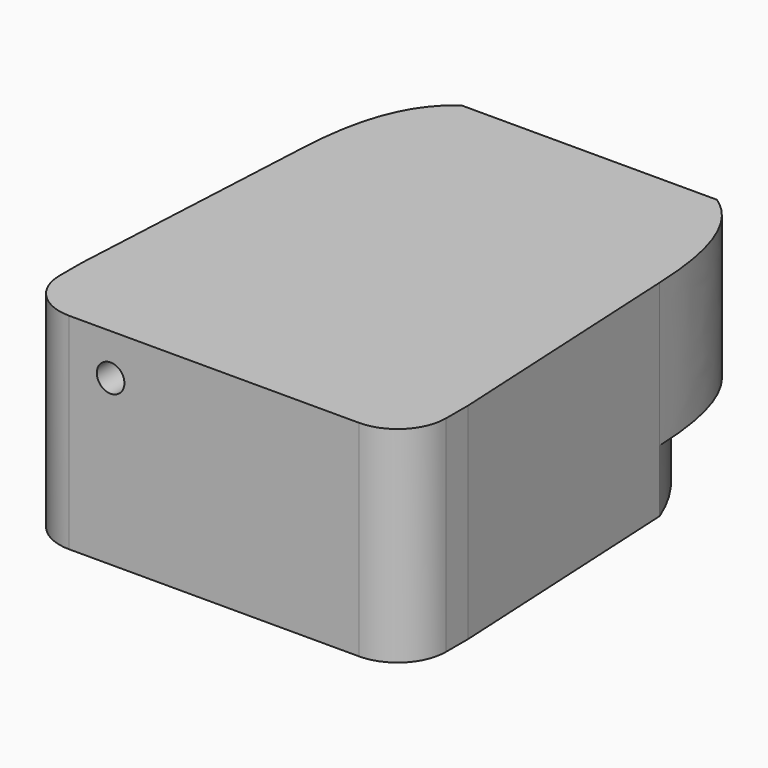
from build123d import *

# Parameters (mm, degrees)
F1_DEPTH  = 4.5
F3_DEPTH  = 10.4
F5_DEPTH  = 13.4
F6_R      = 3.7
F6_R_2    = 1.6
F7_DEPTH  = 5
F8_R      = 1.6
F8_R_2    = 3.7
F9_DEPTH  = 5
F10_R     = 1
F11_DEPTH = 2
F12_W     = 10
F12_H     = 1.5
F13_DEPTH = 3


with BuildPart() as f1:
    # F0 (on Top) → F1 (new body)
    with BuildSketch(Plane.XY):
        with BuildLine():
            ThreePointArc((-14, -13.8007847667), (-12.9748737342, -16.2756585008), (-10.5, -17.3007847667))
            Line((-10.5, -17.3007847667), (-6.75, -17.3007847667))
            Line((-6.75, -17.3007847667), (6.75, -17.3007847667))
            Line((6.75, -17.3007847667), (10.5, -17.3007847667))
            ThreePointArc((10.5, -17.3007847667), (12.9748737342, -16.2756585008), (14, -13.8007847667))
            Line((14, -13.8007847667), (14, -11.8007847667))
            Line((14, -11.8007847667), (13.0486556537, 6.7504299853))
            ThreePointArc((13.0486556537, 6.7504299853), (11.6774697173, 9.4001806183), (9.7759521317, 11.6992152333))
            Line((9.7759521317, 11.6992152333), (-9.7759521317, 11.6992152333))
            ThreePointArc((-9.7759521317, 11.6992152333), (-11.6774697173, 9.4001806183), (-13.0486556537, 6.7504299853))
            Line((-13.0486556537, 6.7504299853), (-14, -11.8007847667))
            Line((-14, -11.8007847667), (-14, -13.8007847667))
        make_face()
    extrude(amount=F1_DEPTH)

    # F2 (on face) → F3 (join)
    with BuildSketch(Plane.XY.offset(4.5)):
        with BuildLine():
            Line((14, -13.8007847667), (14, -11.8007847667))
            Line((14, -11.8007847667), (13.0486556537, 6.7504299853))
            add(Edge.make_bspline(
                [(13.0486556537, 6.7504299853), (12.8450421616, 12.0132155716), (11.5178218111, 15.1653625071), (9.2356767608, 16.6992152333)],
                knots=[0, 0, 0, 0, 10.6544420759, 10.6544420759, 10.6544420759, 10.6544420759], degree=3))
            Line((9.2356767608, 16.6992152333), (-9.2356767608, 16.6992152333))
            add(Edge.make_bspline(
                [(-13.0486556537, 6.7504299853), (-12.8450421616, 12.0132155716), (-11.5178218111, 15.1653625071), (-9.2356767608, 16.6992152333)],
                knots=[0, 0, 0, 0, 10.6544420759, 10.6544420759, 10.6544420759, 10.6544420759], degree=3))
            Line((-13.0486556537, 6.7504299853), (-14, -11.8007847667))
            Line((-14, -11.8007847667), (-14, -13.8007847667))
            ThreePointArc((-14, -13.8007847667), (-12.9748737342, -16.2756585008), (-10.5, -17.3007847667))
            Line((-10.5, -17.3007847667), (10.5, -17.3007847667))
            ThreePointArc((10.5, -17.3007847667), (12.9748737342, -16.2756585008), (14, -13.8007847667))
        make_face()
    extrude(amount=F3_DEPTH)

    # F4 (on face) → F5 (cut)
    with BuildSketch(Plane.XY):
        with BuildLine():
            Line((0, -15.3007847667), (8.5, -15.3007847667))
            ThreePointArc((8.5, -15.3007847667), (10.9748737342, -14.2756585008), (12, -11.8007847667))
            Line((12, -11.8007847667), (12, 5.1777003818))
            ThreePointArc((12, 5.1777003818), (10.8666119051, 7.8556244429), (9.145150881, 10.1992152333))
            Line((9.145150881, 10.1992152333), (-9.145150881, 10.1992152333))
            ThreePointArc((-9.145150881, 10.1992152333), (-10.8666119051, 7.8556244429), (-12, 5.1777003818))
            Line((-12, 5.1777003818), (-12, -11.8007847667))
            ThreePointArc((-12, -11.8007847667), (-10.9748737342, -14.2756585008), (-8.5, -15.3007847667))
            Line((-8.5, -15.3007847667), (0, -15.3007847667))
        make_face()
    extrude(amount=F5_DEPTH, mode=Mode.SUBTRACT)

    # F6 (on face) → F7 (cut)
    with BuildSketch(Plane(origin=(0, 16.6992152333, 0), x_dir=(-1, 0, 0), z_dir=(0, 1, 0))):
        with Locations((-4.6178383804, 9.7)):
            Circle(F6_R)
        with Locations((4.6178383804, 9.7)):
            Circle(F6_R_2)
    extrude(amount=-F7_DEPTH, mode=Mode.SUBTRACT)

    # F8 (on face) → F9 (cut)
    with BuildSketch(Plane.XZ.offset(-10.1992152333)):
        with Locations((4.6178383804, 9.7)):
            Circle(F8_R)
        with Locations((-4.6178383804, 9.7)):
            Circle(F8_R_2)
    extrude(amount=-F9_DEPTH, mode=Mode.SUBTRACT)

    # F10 (on face) → F11 (cut, through all)
    with BuildSketch(Plane.XZ.offset(17.3007847667)):
        with Locations((-7.5, 11.9)):
            Circle(F10_R)
    extrude(amount=-F11_DEPTH, mode=Mode.SUBTRACT)

    # F12 (on face) → F13 (cut)
    with BuildSketch(Plane(origin=(0, 0, 0), x_dir=(1, 0, 0), z_dir=(0, 0, -1))):
        with Locations((0, -10.9492152333)):
            Rectangle(F12_W, F12_H)
    extrude(amount=-F13_DEPTH, mode=Mode.SUBTRACT)


solid = f1.part
